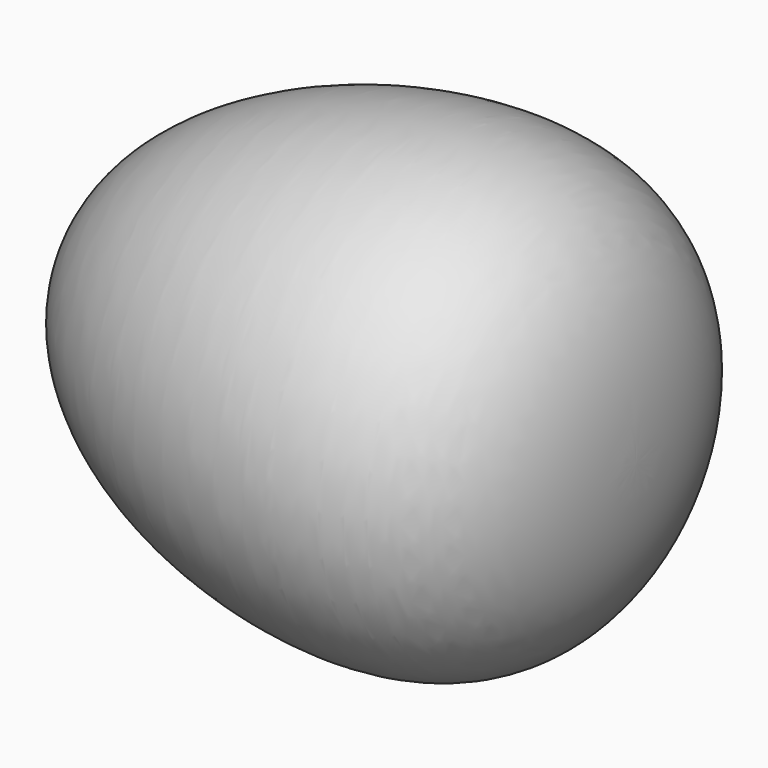
from build123d import *


with BuildPart() as f1:
    # F0 (on Front) → F1 (revolve)
    with BuildSketch(Plane.XZ):
        with BuildLine():
            Line((-60, 0), (0, 0))
            add(Edge.make_bspline(
                [(-60, 0), (-60, 15), (-22.9209910094, 32.2906327967), (0, 20), (0, 0)],
                knots=[0, 0, 0, 0, 0.5244830348, 1, 1, 1, 1], degree=3))
        make_face()
    revolve(axis=Axis((-30, 0, 0), (-1, 0, 0)))


solid = f1.part
